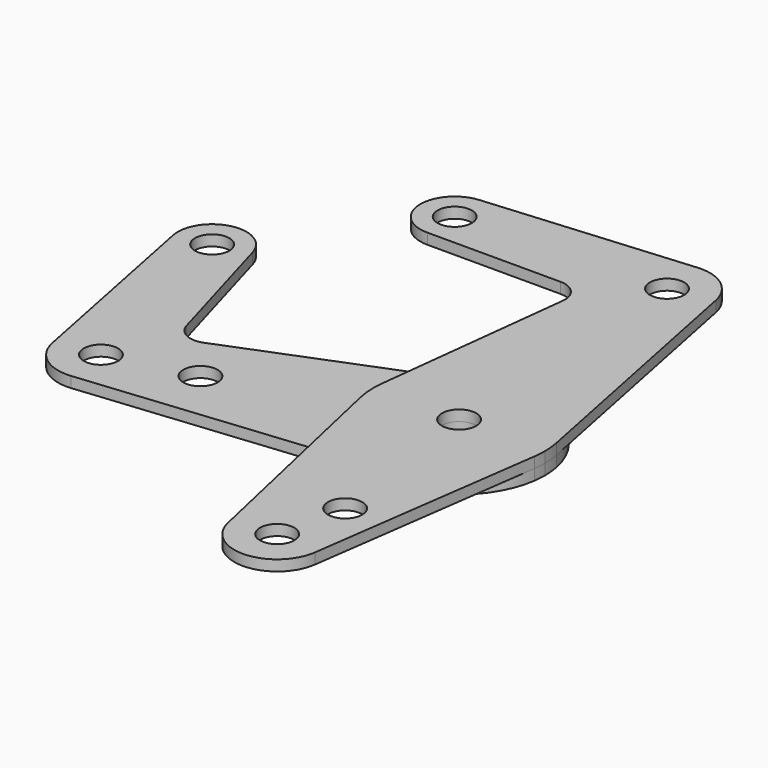
from build123d import *

# Parameters (mm, degrees)
F0_R     = 5.08
F1_DEPTH = 3.175
F2_DEPTH = 3.175


# Not quite as in the source:
# - a feature names something its author has since deleted; it is built from what else it names


with BuildPart() as f1:
    # F0 (on Top) → F1 (new body)
    with BuildSketch(Plane.XY):
        with BuildLine():
            ThreePointArc((10.16, 100.3741442614), (6.8786240281, 107.8514520309), (-0.8459313937, 110.4988664836))
            ThreePointArc((-0.8459313937, 110.4988664836), (-10.1511767243, 99.9508109281), (0, 90.2141442614))
            ThreePointArc((0, 90.2141442614), (7.1842048969, 93.1899393645), (10.16, 100.3741442614))
        make_face()
        with Locations((0, 100.3741442614)):
            Circle(F0_R, mode=Mode.SUBTRACT)
        with BuildLine():
            ThreePointArc((54.8716142506, -52.2704518609), (67.7917463532, -62.174826644), (79.8423690943, -51.229099398))
            ThreePointArc((79.8423690943, -51.229099398), (79.9324913965, -50.3595474809), (79.9625796865, -49.4858557386))
            ThreePointArc((79.9625796865, -49.4858557386), (65.8617336987, -36.8633508161), (54.8716142506, -52.2704518609))
        make_face()
        with Locations((67.2625796865, -49.4858557386)):
            Circle(F0_R, mode=Mode.SUBTRACT)
        with BuildLine():
            ThreePointArc((73.3578412331, 105.4177527176), (73.5446019833, 104.1721352658), (73.6070603461, 102.9141442614))
            ThreePointArc((73.6070603461, 102.9141442614), (52.3087803109, 93.5675095495), (59.849646104, 115.5700470392))
            Line((59.849646104, 115.5700470392), (-0.8459313937, 110.4988664836))
            ThreePointArc((-0.8459313937, 110.4988664836), (6.8786240281, 107.8514520309), (10.16, 100.3741442614))
            ThreePointArc((10.16, 100.3741442614), (7.1842048969, 93.1899393645), (0, 90.2141442614))
            Line((0, 90.2141442614), (39.5282835187, 90.2141442614))
            ThreePointArc((39.5282835187, 90.2141442614), (44.2691931384, 88.0886295528), (45.8362844499, 83.135018585))
            Line((45.8362844499, 83.135018585), (40.8079958174, 39.6329853928))
            Line((40.8079958174, 39.6329853928), (54.917810899, 45.2391646928))
            ThreePointArc((54.917810899, 45.2391646928), (76.4089843694, 43.9601796602), (89.1982324351, 26.6413611739))
            Line((89.1982324351, 26.6413611739), (73.3578412331, 105.4177527176))
        make_face()
        with BuildLine():
            ThreePointArc((39.0646669362, 24.550646967), (44.1352803506, 37.083362389), (54.917810899, 45.2391646928))
            Line((54.917810899, 45.2391646928), (40.8079958174, 39.6329853928))
            Line((40.8079958174, 39.6329853928), (39.0646669362, 24.550646967))
        make_face()
        with BuildLine():
            Line((44.4451075952, -5.8743218991), (66.8202917314, -3.6401774247))
            ThreePointArc((66.8202917314, -3.6401774247), (49.4329187665, 1.0373270408), (39.514739789, 16.0649520167))
            Line((39.514739789, 16.0649520167), (44.4451075952, -5.8743218991))
        make_face()
        with BuildLine():
            ThreePointArc((59.849646104, 115.5700470392), (52.3087803109, 93.5675095495), (73.6070603461, 102.9141442614))
            ThreePointArc((73.6070603461, 102.9141442614), (73.5446019833, 104.1721352658), (73.3578412331, 105.4177527176))
            ThreePointArc((73.3578412331, 105.4177527176), (68.5372288157, 113.0665099525), (59.849646104, 115.5700470392))
        make_face()
        with Locations((60.9070603461, 102.9141442614)):
            Circle(F0_R, mode=Mode.SUBTRACT)
        with BuildLine():
            Line((79.8423690943, -51.229099398), (89.4562494765, 18.1476569426))
            ThreePointArc((89.4562494765, 18.1476569426), (81.9110772813, 3.3340710535), (66.8202917314, -3.6401774247))
            Line((66.8202917314, -3.6401774247), (44.4451075952, -5.8743218991))
            Line((44.4451075952, -5.8743218991), (54.8716142506, -52.2704518609))
            ThreePointArc((54.8716142506, -52.2704518609), (65.8617336987, -36.8633508161), (79.9625796865, -49.4858557386))
            ThreePointArc((79.9625796865, -49.4858557386), (79.9324913965, -50.3595474809), (79.8423690943, -51.229099398))
        make_face()
        with Locations((71.5183865738, -29.616519873)):
            Circle(F0_R, mode=Mode.SUBTRACT)
        with BuildLine():
            ThreePointArc((89.696670661, 21.6341442614), (89.5717539355, 24.1501262702), (89.1982324351, 26.6413611739))
            ThreePointArc((89.1982324351, 26.6413611739), (76.4089843694, 43.9601796602), (54.917810899, 45.2391646928))
            ThreePointArc((54.917810899, 45.2391646928), (44.1352803506, 37.083362389), (39.0646669362, 24.550646967))
            ThreePointArc((39.0646669362, 24.550646967), (38.9323222925, 20.288844354), (39.514739789, 16.0649520167))
            ThreePointArc((39.514739789, 16.0649520167), (49.4329187665, 1.0373270408), (66.8202917314, -3.6401774247))
            ThreePointArc((66.8202917314, -3.6401774247), (81.9110772813, 3.3340710535), (89.4562494765, 18.1476569426))
            ThreePointArc((89.4562494765, 18.1476569426), (89.636494081, 19.8867607767), (89.696670661, 21.6341442614))
        make_face()
        with Locations((64.296670661, 21.6341442614)):
            Circle(F0_R, mode=Mode.SUBTRACT)
    extrude(amount=F1_DEPTH)


with BuildPart() as f2:
    # F0 (on Top) → F2 (new body)
    with BuildSketch(Plane.XY):
        with BuildLine():
            ThreePointArc((-28.8099856228, 59.2292622952), (-28.9097724352, 60.6497237067), (-29.207172753, 62.0422828905))
            ThreePointArc((-29.207172753, 62.0422828905), (-41.3737794296, 69.1008060111), (-48.9331146431, 57.2388703429))
            ThreePointArc((-48.9331146431, 57.2388703429), (-37.9699333358, 49.1185998331), (-28.8099856228, 59.2292622952))
        make_face()
        with Locations((-38.9699856228, 59.2292622952)):
            Circle(F0_R, mode=Mode.SUBTRACT)
        with BuildLine():
            ThreePointArc((-37.0011340573, -2.4879899404), (-32.1015061527, -10.2089569865), (-23.2854122466, -12.6371608431))
            ThreePointArc((-23.2854122466, -12.6371608431), (-15.1314117759, -8.5224704811), (-11.8472227818, 0))
            ThreePointArc((-11.8472227818, 0), (-25.7972881405, 12.6383280777), (-37.0011340573, -2.4879899404))
        make_face()
        with Locations((-24.5472227818, 0)):
            Circle(F0_R, mode=Mode.SUBTRACT)
        with BuildLine():
            ThreePointArc((39.0646669362, 24.550646967), (44.1352803506, 37.083362389), (54.917810899, 45.2391646928))
            Line((54.917810899, 45.2391646928), (40.8079958174, 39.6329853928))
            Line((40.8079958174, 39.6329853928), (39.0646669362, 24.550646967))
        make_face()
        with BuildLine():
            Line((44.4451075952, -5.8743218991), (66.8202917314, -3.6401774247))
            ThreePointArc((66.8202917314, -3.6401774247), (49.4329187665, 1.0373270408), (39.514739789, 16.0649520167))
            Line((39.514739789, 16.0649520167), (44.4451075952, -5.8743218991))
        make_face()
        with BuildLine():
            ThreePointArc((89.696670661, 21.6341442614), (89.5717539355, 24.1501262702), (89.1982324351, 26.6413611739))
            ThreePointArc((89.1982324351, 26.6413611739), (76.4089843694, 43.9601796602), (54.917810899, 45.2391646928))
            ThreePointArc((54.917810899, 45.2391646928), (44.1352803506, 37.083362389), (39.0646669362, 24.550646967))
            ThreePointArc((39.0646669362, 24.550646967), (38.9323222925, 20.288844354), (39.514739789, 16.0649520167))
            ThreePointArc((39.514739789, 16.0649520167), (49.4329187665, 1.0373270408), (66.8202917314, -3.6401774247))
            ThreePointArc((66.8202917314, -3.6401774247), (81.9110772813, 3.3340710535), (89.4562494765, 18.1476569426))
            ThreePointArc((89.4562494765, 18.1476569426), (89.636494081, 19.8867607767), (89.696670661, 21.6341442614))
        make_face()
        with Locations((64.296670661, 21.6341442614)):
            Circle(F0_R, mode=Mode.SUBTRACT)
        with BuildLine():
            ThreePointArc((39.514739789, 16.0649520167), (38.9323222925, 20.288844354), (39.0646669362, 24.550646967))
            Line((39.0646669362, 24.550646967), (40.8079958174, 39.6329853928))
            Line((40.8079958174, 39.6329853928), (-9.7136466081, 19.5594844768))
            ThreePointArc((-9.7136466081, 19.5594844768), (-14.8548233, 19.7596605926), (-18.1601195922, 23.7026017126))
            Line((-18.1601195922, 23.7026017126), (-29.207172753, 62.0422828905))
            ThreePointArc((-29.207172753, 62.0422828905), (-28.9097724352, 60.6497237067), (-28.8099856228, 59.2292622952))
            ThreePointArc((-28.8099856228, 59.2292622952), (-37.9699333358, 49.1185998331), (-48.9331146431, 57.2388703429))
            Line((-48.9331146431, 57.2388703429), (-37.0011340573, -2.4879899404))
            ThreePointArc((-37.0011340573, -2.4879899404), (-25.7972881405, 12.6383280777), (-11.8472227818, 0))
            ThreePointArc((-11.8472227818, 0), (-15.1314117759, -8.5224704811), (-23.2854122466, -12.6371608431))
            Line((-23.2854122466, -12.6371608431), (44.4451075952, -5.8743218991))
            Line((44.4451075952, -5.8743218991), (39.514739789, 16.0649520167))
        make_face()
        with Locations((0.1316365078, 6.0094845171)):
            Circle(F0_R, mode=Mode.SUBTRACT)
    extrude(amount=-F2_DEPTH)


solid = Compound([f1.part, f2.part])
